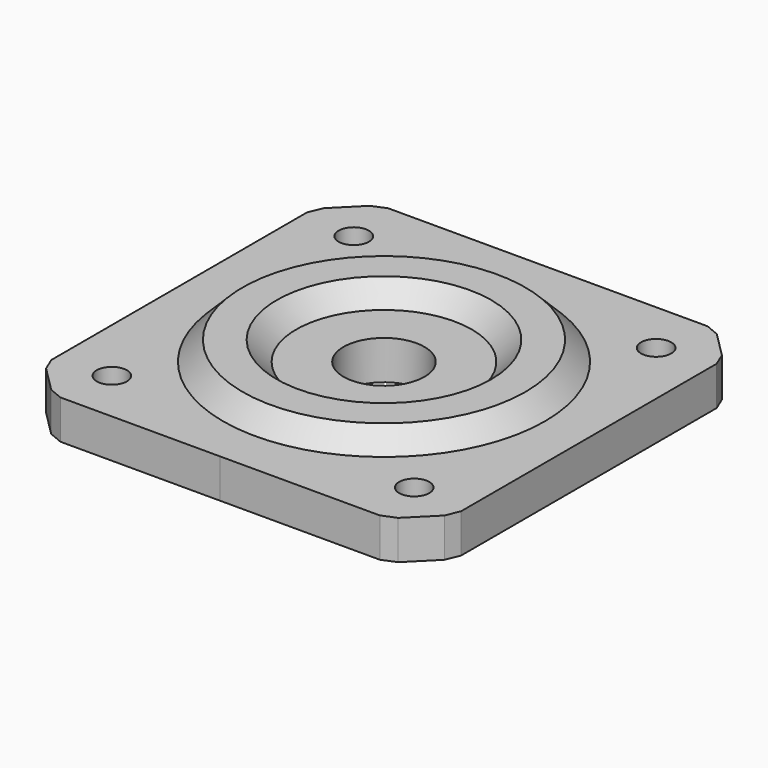
from build123d import *

# Parameters (mm, degrees)
F0_R     = 1.55
F0_R_2   = 16.5
F0_R_3   = 11.0000000003
F0_R_4   = 4.1499999994
F1_DEPTH = 4
F2_R     = 16.5
F2_R_2   = 11.0000000003
F3_DEPTH = 2
F4_SIZE  = 1.99999
F5_SIZE  = 1.99999


# Not quite as in the source:
# - a fillet or chamfer is up to 0.001 mm smaller than in the source, because OpenCascade refuses the exact size


with BuildPart() as f1:
    # F0 (on Top) → F1 (new body)
    with BuildSketch(Plane.XY):
        Polygon((10.9770673246, 19.3054056901), (-5.3945055504, 19.3054056901), (-21.7660784254, 19.3054056904), (-23.1802919884, 18.7196192521), (-25.8087191127, 16.0911921274), (-26.3945055504, 14.6769785651), (-26.3945055504, -18.0661671849), (-25.8087191127, -19.4803807472), (-23.1802919884, -22.1088078719), (-21.7660784254, -22.6945943101), (-5.3945055504, -22.6945943099), (10.9770673246, -22.6945943084), (12.3912808869, -22.1088078705), (15.0197080109, -19.4803807465), (15.6054944488, -18.0661671842), (15.6054944488, 14.6769785659), (15.0197080109, 16.0911921281), (12.3912808869, 18.7196192521), align=None)
        with Locations((-20.8945055404, -17.1945943099)):
            Circle(F0_R, mode=Mode.SUBTRACT)
        with Locations((-5.3945055504, -1.6945943099)):
            Circle(F0_R_2, mode=Mode.SUBTRACT)
        with Locations((10.1054944396, -17.1945943099)):
            Circle(F0_R, mode=Mode.SUBTRACT)
        with Locations((-20.8945055501, 13.8054056901)):
            Circle(F0_R, mode=Mode.SUBTRACT)
        with Locations((10.1054944396, 13.8054056901)):
            Circle(F0_R, mode=Mode.SUBTRACT)
        with Locations((-5.3945055504, -1.6945943099)):
            Circle(F0_R_2)
        with Locations((-5.3945055504, -1.6945943099)):
            Circle(F0_R_3, mode=Mode.SUBTRACT)
        with Locations((-5.3945055504, -1.6945943099)):
            Circle(F0_R_3)
        with Locations((-5.3945055504, -1.6945943099)):
            Circle(F0_R_4, mode=Mode.SUBTRACT)
    extrude(amount=F1_DEPTH)

    # F2 (on face) → F3 (join)
    with BuildSketch(Plane.XY.offset(4)):
        with Locations((-5.3945055504, -1.6945943099)):
            Circle(F2_R)
        with Locations((-5.3945055504, -1.6945943099)):
            Circle(F2_R_2, mode=Mode.SUBTRACT)
    extrude(amount=F3_DEPTH)

    # F4 (size 2 in the source; OpenCascade refuses exactly that, so slightly less here)
    f4_edges = [f1.edges().sort_by_distance(p)[0] for p in [
        (-21.894506, -1.694594, 6),
    ]]
    chamfer(f4_edges, length=F4_SIZE)

    # F5 (size 2 in the source; OpenCascade refuses exactly that, so slightly less here)
    f5_edges = [f1.edges().sort_by_distance(p)[0] for p in [
        (-16.394506, -1.694594, 4),
    ]]
    chamfer(f5_edges, length=F5_SIZE)


solid = f1.part
